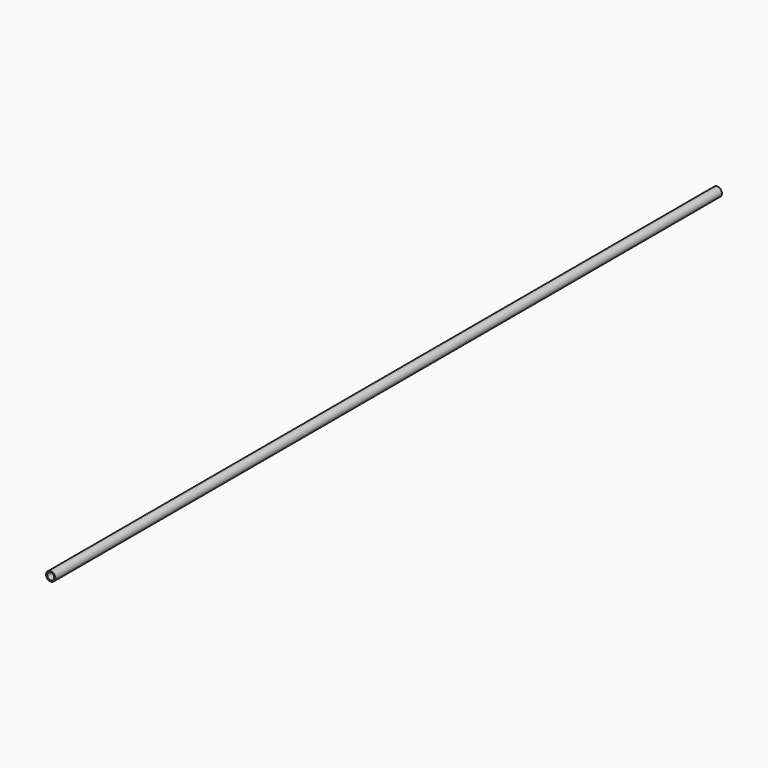
from build123d import *

# Parameters (mm, degrees)
F0_R          = 9.525
F0_R_2        = 7.14375
F1_DEPTH      = 855.98
F1_DEPTH_BACK = 855.98


# Not quite as in the source:
# - a feature names something its author has since deleted; it is built from what else it names


with BuildPart() as f1:
    # F0 (on Front) → F1 (new body, two sides)
    with BuildSketch(Plane.XZ) as f1_sk:
        Circle(F0_R)
        Circle(F0_R_2, mode=Mode.SUBTRACT)
    extrude(amount=F1_DEPTH)
    extrude(f1_sk.sketch, amount=-F1_DEPTH_BACK)


solid = f1.part
